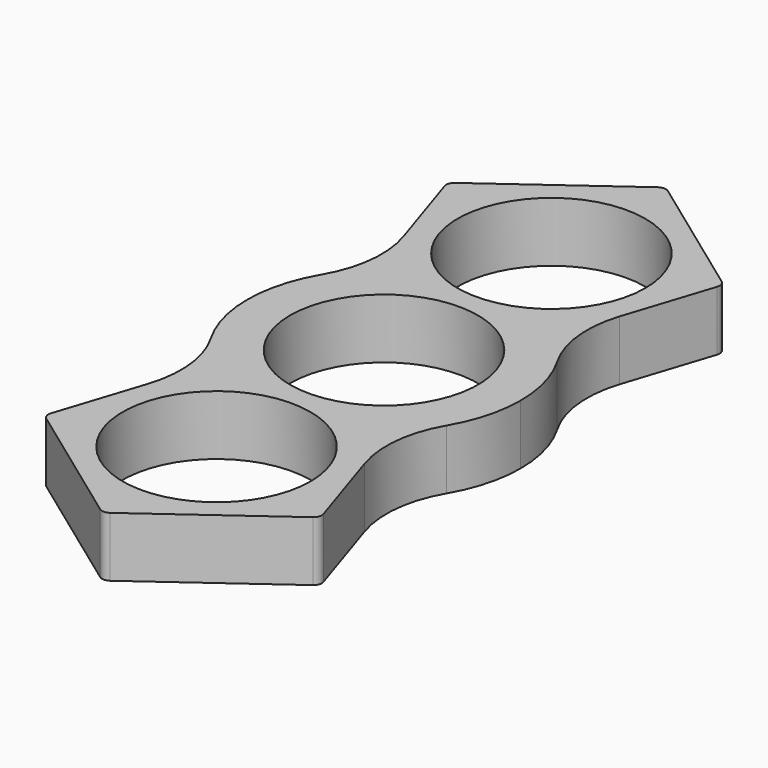
from build123d import *
from build123d import SkipClean  # not in build123d's __all__

# Parameters (mm, degrees)
F1_DEPTH = 3.5
F3_R     = 11
F4_DEPTH = 7.001


with BuildPart() as f1:
    # F0 (on Top) → F1 (new body, symmetric)
    with BuildSketch(Plane.XY):
        with BuildLine():
            ThreePointArc((-11, 0), (0, 11), (11, 0))
            Line((11, 0), (16, 0))
            ThreePointArc((16, 0), (15.4421025537, 4.1882536601), (13.8073164099, 8.0844303175))
            ThreePointArc((13.8073164099, 8.0844303175), (12.1011838507, 13.2547074929), (12.6620262811, 18.6702508773))
            Line((12.6620262811, 18.6702508773), (15.9510565163, 28.7928450855))
            ThreePointArc((15.9510565163, 28.7928450855), (15.9510565163, 29.4108790743), (15.5877852523, 29.9108790743))
            Line((15.5877852523, 29.9108790743), (0.5877852523, 40.8090169944))
            ThreePointArc((0.5877852523, 40.8090169944), (0, 41), (-0.5877852523, 40.8090169944))
            Line((-0.5877852523, 40.8090169944), (-15.5877852523, 29.9108790743))
            ThreePointArc((-15.5877852523, 29.9108790743), (-15.9510565163, 29.4108790743), (-15.9510565163, 28.7928450855))
            Line((-15.9510565163, 28.7928450855), (-12.6620262811, 18.6702508773))
            ThreePointArc((-12.6620262811, 18.6702508773), (-12.1011838507, 13.2547074929), (-13.8073164099, 8.0844303175))
            ThreePointArc((-13.8073164099, 8.0844303175), (-15.4421025537, 4.1882536601), (-16, 0))
            Line((-16, 0), (-11, 0))
        make_face()
    extrude(amount=F1_DEPTH, both=True)

    # F2: F1 across face


with BuildPart() as f1_1:
    add(f1.part, clean=False)
    with SkipClean():  # cleaning this boolean's faces spoils the solid; the shape is the same uncleaned
        add(f1.part.mirror(Plane(origin=(-13.5, 0, 0), x_dir=(1, 0, 0), z_dir=(0, -1, 0))), clean=False)

    # F3 (on face) → F4 (cut, through all)
    with BuildSketch(Plane.XY.offset(3.5)):
        with Locations((0, 24.5)):
            Circle(F3_R)
        with Locations((0, -24.5)):
            Circle(F3_R)
    extrude(amount=-F4_DEPTH, mode=Mode.SUBTRACT)


solid = f1_1.part
